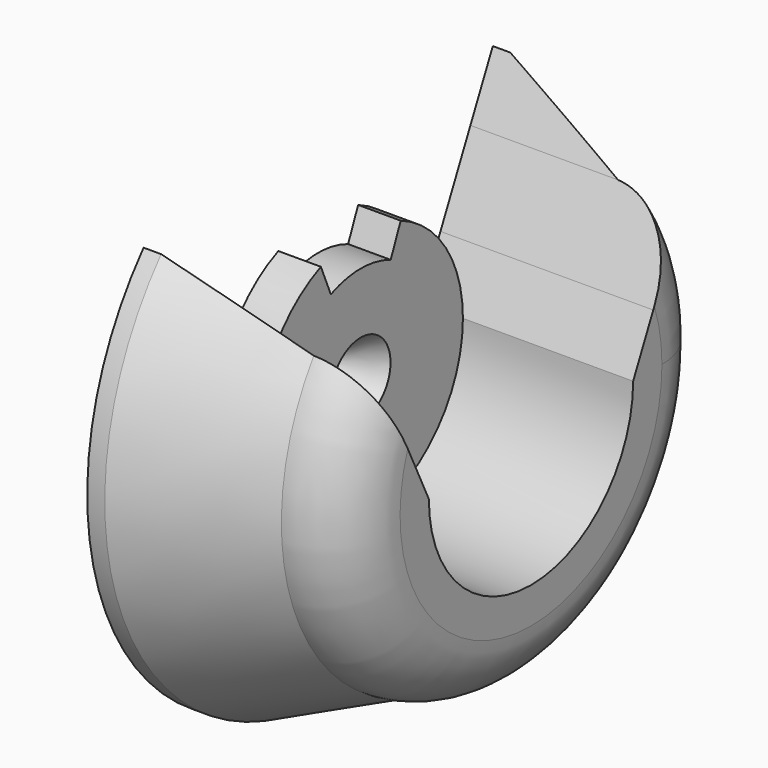
from build123d import *

# Parameters (mm, degrees)
F1_DEPTH       = 20
F2_DEPTH       = 20
F3_R           = 6.3
F4_DEPTH       = 14
F5_S5_R        = 21.6830909865
F5_T6_DEPTH    = 40
F6_DEPTH       = 4
F7_DEPTH       = 25
F9_D           = 2.7
F9_DEPTH       = 12
F9_CSINK_D     = 7
F9_CSINK_ANGLE = 66
F9_TIP         = 0.8111618357


# Not quite as in the source:
# - a fillet or chamfer that OpenCascade refuses, or shapes differently, is made with other operations: its cross-section is extruded or revolved along the edge and cut away or added


with BuildPart() as f1:
    # F0 (on Right) → F1 (new body)
    with BuildSketch(Plane.YZ):
        with BuildLine():
            ThreePointArc((4.6887735419, 11.0460582414), (10.0066298648, 6.6232438237), (12, 0))
            Line((12, 0), (14.3613430429, 4.925409334))
            ThreePointArc((14.3613430429, 4.925409334), (0, 15.1824843522), (-14.3613430429, 4.925409334))
            Line((-14.3613430429, 4.925409334), (-12, 0))
            ThreePointArc((-12, 0), (-10.0066298648, 6.6232438237), (-4.6887735419, 11.0460582414))
            ThreePointArc((-4.6887735419, 11.0460582414), (0, 12), (4.6887735419, 11.0460582414))
        make_face()
        with BuildLine():
            Line((14.3613430429, 4.925409334), (12, 0))
            ThreePointArc((12, 0), (0, -12), (-12, 0))
            Line((-12, 0), (-14.3613430429, 4.925409334))
            ThreePointArc((-14.3613430429, 4.925409334), (-2.4966943224, -14.9757920847), (15.1824843522, 0))
            ThreePointArc((15.1824843522, 0), (14.9757920847, 2.4966943224), (14.3613430429, 4.925409334))
        make_face()
    extrude(amount=F1_DEPTH)

    # F0 (on Right) → F2 (join)
    with BuildSketch(Plane.YZ):
        with BuildLine():
            ThreePointArc((-14.3613430429, 4.925409334), (0, 15.1824843522), (14.3613430429, 4.925409334))
            Line((14.3613430429, 4.925409334), (17.8804215677, 12.2656821778))
            ThreePointArc((17.8804215677, 12.2656821778), (13.0689294726, 17.30200905), (6.9088656071, 20.5529562533))
            Line((6.9088656071, 20.5529562533), (-6.9088656071, 20.5529562533))
            ThreePointArc((-6.9088656071, 20.5529562533), (-13.0689294726, 17.30200905), (-17.8804215677, 12.2656821778))
            Line((-17.8804215677, 12.2656821778), (-14.3613430429, 4.925409334))
        make_face()
        with BuildLine():
            Line((17.8804215677, 12.2656821778), (14.3613430429, 4.925409334))
            ThreePointArc((14.3613430429, 4.925409334), (14.9757920847, 2.4966943224), (15.1824843522, 0))
            ThreePointArc((15.1824843522, 0), (-2.4966943224, -14.9757920847), (-14.3613430429, 4.925409334))
            Line((-14.3613430429, 4.925409334), (-17.8804215677, 12.2656821778))
            ThreePointArc((-17.8804215677, 12.2656821778), (-6.4208109689, -20.710616148), (21.6830909865, 0))
            ThreePointArc((21.6830909865, 0), (20.710616148, 6.4208109689), (17.8804215677, 12.2656821778))
        make_face()
        with BuildLine():
            Line((-6.9088656071, 20.5529562533), (6.9088656071, 20.5529562533))
            ThreePointArc((6.9088656071, 20.5529562533), (0, 21.6830909865), (-6.9088656071, 20.5529562533))
        make_face()
    extrude(amount=F2_DEPTH)

    # F3
    f3_edges = [f1.edges().sort_by_distance(p)[0] for p in [
        (20, -6.908866, -20.552956),
    ]]
    fillet(f3_edges, radius=F3_R)

    # F0 (on Right) → F4 (join)
    with BuildSketch(Plane.YZ):
        with BuildLine():
            ThreePointArc((6.9088656071, 20.5529562533), (13.0689294726, 17.30200905), (17.8804215677, 12.2656821778))
            Line((17.8804215677, 12.2656821778), (20.5131543573, 17.7571700385))
            ThreePointArc((20.5131543573, 17.7571700385), (19.1631742939, 19.2062318127), (17.7110863222, 20.5529562533))
            Line((17.7110863222, 20.5529562533), (6.9088656071, 20.5529562533))
        make_face()
        with BuildLine():
            ThreePointArc((-6.9088656071, 20.5529562533), (0, 21.6830909865), (6.9088656071, 20.5529562533))
            Line((6.9088656071, 20.5529562533), (17.7110863222, 20.5529562533))
            ThreePointArc((17.7110863222, 20.5529562533), (0, 27.1312843312), (-17.7110863222, 20.5529562533))
            Line((-17.7110863222, 20.5529562533), (-6.9088656071, 20.5529562533))
        make_face()
        with BuildLine():
            Line((-20.5131543573, 17.7571700385), (-17.8804215677, 12.2656821778))
            ThreePointArc((-17.8804215677, 12.2656821778), (-13.0689294726, 17.30200905), (-6.9088656071, 20.5529562533))
            Line((-6.9088656071, 20.5529562533), (-17.7110863222, 20.5529562533))
            ThreePointArc((-17.7110863222, 20.5529562533), (-19.1631742939, 19.2062318127), (-20.5131543573, 17.7571700385))
        make_face()
        with BuildLine():
            Line((20.5131543573, 17.7571700385), (17.8804215677, 12.2656821778))
            ThreePointArc((17.8804215677, 12.2656821778), (20.710616148, 6.4208109689), (21.6830909865, 0))
            ThreePointArc((21.6830909865, 0), (-6.4208109689, -20.710616148), (-17.8804215677, 12.2656821778))
            Line((-17.8804215677, 12.2656821778), (-20.5131543573, 17.7571700385))
            ThreePointArc((-20.5131543573, 17.7571700385), (-9.4751877571, -25.4229700552), (27.1312843312, 0))
            ThreePointArc((27.1312843312, 0), (25.4229700552, 9.4751877571), (20.5131543573, 17.7571700385))
        make_face()
    extrude(amount=F4_DEPTH)

    # F5: chamfer of 5.5 x 12.3532022565 on 1 edges, made by hand


with BuildPart() as f5_tool2:
    # F5_s3 → F5_t4 (revolve)
    with BuildSketch(Plane(origin=(0, 0, 0), x_dir=(1, 0, 0), z_dir=(0, 0.6544905808, 0.7560701553))):
        Polygon((14, -21.6312843312), (1.6467977435, -27.1312843312), (14, -27.1312843312), align=None)
    revolve(axis=Axis((14, 0, 0), (1, 0, 0)))

    # F5_s5 → F5_t6 (cut, symmetric)
    with BuildSketch(Plane.YZ.offset(7.8)):
        Circle(F5_S5_R)
    extrude(amount=F5_T6_DEPTH, both=True, mode=Mode.SUBTRACT)


with BuildPart() as f1_1:
    add(f1.part)

    # F5_t1: cut F5_tool2
    add(f5_tool2.part, mode=Mode.SUBTRACT)

    # F0 (on Right) → F6 (join)
    with BuildSketch(Plane.YZ):
        with BuildLine():
            ThreePointArc((-12, 0), (0, -12), (12, 0))
            ThreePointArc((12, 0), (10.0066298648, 6.6232438237), (4.6887735419, 11.0460582414))
            Line((4.6887735419, 11.0460582414), (3.5165801564, 8.2845436811))
            ThreePointArc((3.5165801564, 8.2845436811), (7.5049723986, 4.9674328678), (9, 0))
            ThreePointArc((9, 0), (-4.9674328678, -7.5049723986), (-3.5165801564, 8.2845436811))
            Line((-3.5165801564, 8.2845436811), (-4.6887735419, 11.0460582414))
            ThreePointArc((-4.6887735419, 11.0460582414), (-10.0066298648, 6.6232438237), (-12, 0))
        make_face()
        with BuildLine():
            ThreePointArc((9, 0), (7.5049723986, 4.9674328678), (3.5165801564, 8.2845436811))
            Line((3.5165801564, 8.2845436811), (0, 0))
            Line((0, 0), (-3.5165801564, 8.2845436811))
            ThreePointArc((-3.5165801564, 8.2845436811), (-4.9674328678, -7.5049723986), (9, 0))
        make_face()
        with BuildLine():
            Line((0, 0), (3.5165801564, 8.2845436811))
            ThreePointArc((3.5165801564, 8.2845436811), (0, 9), (-3.5165801564, 8.2845436811))
            Line((-3.5165801564, 8.2845436811), (0, 0))
        make_face()
    extrude(amount=F6_DEPTH)

    # F0 (on Right) → F7 (cut)
    with BuildSketch(Plane.YZ):
        with BuildLine():
            ThreePointArc((4.6887735419, 11.0460582414), (10.0066298648, 6.6232438237), (12, 0))
            Line((12, 0), (14.3613430429, 4.925409334))
            ThreePointArc((14.3613430429, 4.925409334), (0, 15.1824843522), (-14.3613430429, 4.925409334))
            Line((-14.3613430429, 4.925409334), (-12, 0))
            ThreePointArc((-12, 0), (-10.0066298648, 6.6232438237), (-4.6887735419, 11.0460582414))
            ThreePointArc((-4.6887735419, 11.0460582414), (0, 12), (4.6887735419, 11.0460582414))
        make_face()
        with BuildLine():
            ThreePointArc((-14.3613430429, 4.925409334), (0, 15.1824843522), (14.3613430429, 4.925409334))
            Line((14.3613430429, 4.925409334), (17.8804215677, 12.2656821778))
            ThreePointArc((17.8804215677, 12.2656821778), (13.0689294726, 17.30200905), (6.9088656071, 20.5529562533))
            Line((6.9088656071, 20.5529562533), (-6.9088656071, 20.5529562533))
            ThreePointArc((-6.9088656071, 20.5529562533), (-13.0689294726, 17.30200905), (-17.8804215677, 12.2656821778))
            Line((-17.8804215677, 12.2656821778), (-14.3613430429, 4.925409334))
        make_face()
        with BuildLine():
            Line((-6.9088656071, 20.5529562533), (6.9088656071, 20.5529562533))
            ThreePointArc((6.9088656071, 20.5529562533), (0, 21.6830909865), (-6.9088656071, 20.5529562533))
        make_face()
        with BuildLine():
            ThreePointArc((-6.9088656071, 20.5529562533), (0, 21.6830909865), (6.9088656071, 20.5529562533))
            Line((6.9088656071, 20.5529562533), (17.7110863222, 20.5529562533))
            ThreePointArc((17.7110863222, 20.5529562533), (0, 27.1312843312), (-17.7110863222, 20.5529562533))
            Line((-17.7110863222, 20.5529562533), (-6.9088656071, 20.5529562533))
        make_face()
        with BuildLine():
            Line((-20.5131543573, 17.7571700385), (-17.8804215677, 12.2656821778))
            ThreePointArc((-17.8804215677, 12.2656821778), (-13.0689294726, 17.30200905), (-6.9088656071, 20.5529562533))
            Line((-6.9088656071, 20.5529562533), (-17.7110863222, 20.5529562533))
            ThreePointArc((-17.7110863222, 20.5529562533), (-19.1631742939, 19.2062318127), (-20.5131543573, 17.7571700385))
        make_face()
        with BuildLine():
            ThreePointArc((6.9088656071, 20.5529562533), (13.0689294726, 17.30200905), (17.8804215677, 12.2656821778))
            Line((17.8804215677, 12.2656821778), (20.5131543573, 17.7571700385))
            ThreePointArc((20.5131543573, 17.7571700385), (19.1631742939, 19.2062318127), (17.7110863222, 20.5529562533))
            Line((17.7110863222, 20.5529562533), (6.9088656071, 20.5529562533))
        make_face()
    extrude(amount=F7_DEPTH, mode=Mode.SUBTRACT)

    # F9
    with Locations(Plane.YZ.offset(4)):
        with Locations((0, -0.2123973536)):
            CounterSinkHole(F9_D / 2, F9_CSINK_D / 2, depth=F9_DEPTH, counter_sink_angle=F9_CSINK_ANGLE)
            with Locations((0, 0, -(F9_DEPTH + F9_TIP / 2))):  # 118° drill point
                Cone(0, F9_D / 2, F9_TIP, mode=Mode.SUBTRACT)


solid = f1_1.part
